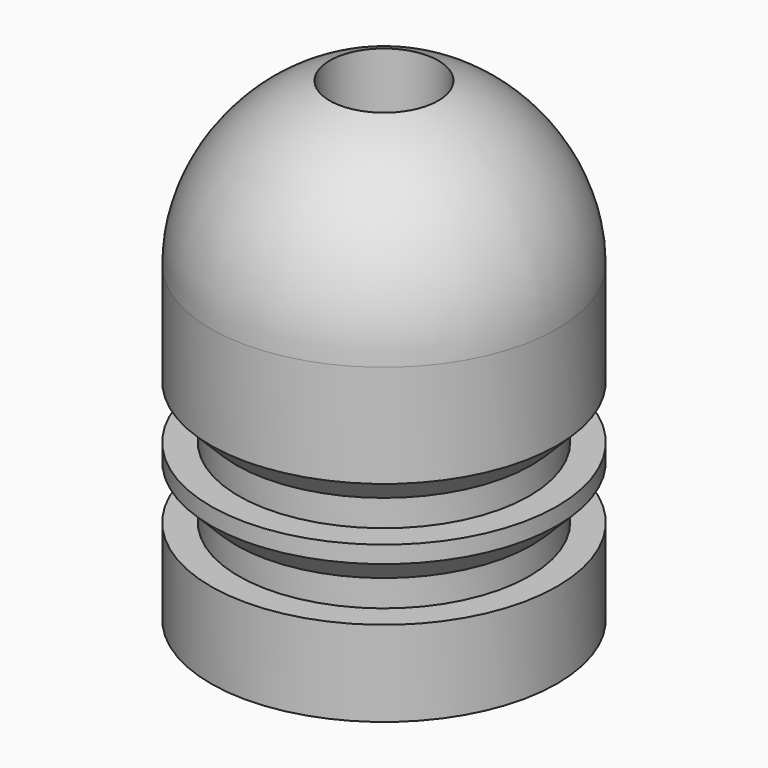
from build123d import *

# Parameters (mm, degrees)
F0_R      = 20.25
F1_DEPTH  = 10
F2_R      = 17
F3_DEPTH  = 3.25
F4_R      = 20.25
F4_R_2    = 17
F5_DEPTH  = 5
F6_R      = 17
F7_DEPTH  = 3.25
F8_R      = 20.25
F8_R_2    = 17
F9_DEPTH  = 25
F10_DEPTH = 5
F11_DEPTH = 5
F13_R     = 6.35
F13_R_2   = 0.25
F14_DEPTH = 20
F15_SIZE  = 3


# Not quite as in the source:
# - a fillet or chamfer that OpenCascade refuses, or shapes differently, is made with other operations: its cross-section is extruded or revolved along the edge and cut away or added


with BuildPart() as f1:
    # F0 (on Top) → F1 (new body)
    with BuildSketch(Plane.XY):
        Circle(F0_R)
    extrude(amount=F1_DEPTH)

    # F2 (on face) → F3 (join)
    with BuildSketch(Plane.XY.offset(10)):
        Circle(F2_R)
    extrude(amount=F3_DEPTH)

    # F4 (on face) → F5 (join)
    with BuildSketch(Plane.XY.offset(13.25)):
        Circle(F4_R)
        Circle(F4_R_2, mode=Mode.SUBTRACT)
        Circle(F4_R_2)
    extrude(amount=F5_DEPTH)

    # F6 (on face) → F7 (join)
    with BuildSketch(Plane.XY.offset(18.25)):
        Circle(F6_R)
    extrude(amount=F7_DEPTH)

    # F8 (on face) → F9 (join)
    with BuildSketch(Plane.XY.offset(21.5)):
        Circle(F8_R)
        Circle(F8_R_2, mode=Mode.SUBTRACT)
        Circle(F8_R_2)
    extrude(amount=F9_DEPTH)

    # F10 (add): a face of the model
    f10_faces = [f1.faces().sort_by_distance(p)[0] for p in [
        (0, 0, 46.5),
    ]]
    extrude(f10_faces, amount=F10_DEPTH)

    # F11 (add): a face of the model
    f11_faces = [f1.faces().sort_by_distance(p)[0] for p in [
        (0, 0, 51.5),
    ]]
    extrude(f11_faces, amount=F11_DEPTH)

    # F12: fillet of radius 20 on 1 edges, made by hand

    # F12_s1 → F12_t2 (revolve, cut)
    with BuildSketch(Plane.XZ):
        with BuildLine():
            add(Edge.make_bspline(
                [(20.25, 36.5), (20.25, 56.5), (0.25, 56.5)],
                knots=[0, 0, 0, 1, 1, 1], degree=2, weights=[1, 0.6666666667, 1]))
            Line((0.25, 56.5), (20.25, 56.5))
            Line((20.25, 56.5), (20.25, 36.5))
        make_face()
    revolve(axis=Axis((0, 0, 56.5), (0, 0, 1)), mode=Mode.SUBTRACT)

    # F13 (on face) → F14 (cut)
    with BuildSketch(Plane.XY.offset(56.5)):
        Circle(F13_R)
        Circle(F13_R_2, mode=Mode.SUBTRACT)
        Circle(F13_R_2)
    extrude(amount=-F14_DEPTH, mode=Mode.SUBTRACT)

    # F15
    f15_edges = [f1.edges().sort_by_distance(p)[0] for p in [
        (-20.25, 0, 13.25),
        (-20.25, 0, 21.5),
    ]]
    chamfer(f15_edges, length=F15_SIZE)


solid = f1.part
